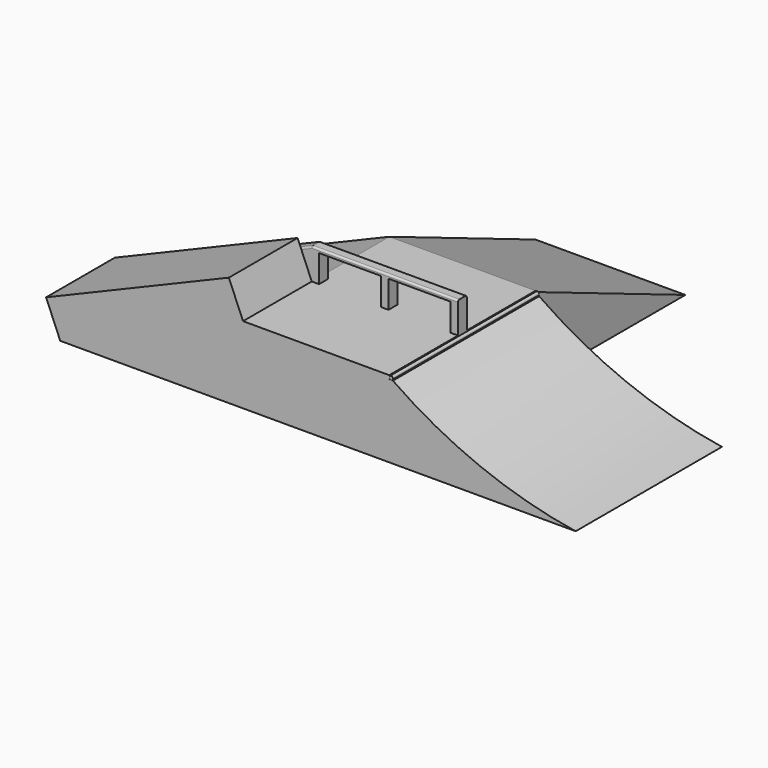
from build123d import *

# Parameters (mm, degrees)
F1_DEPTH     = 127
F2_W         = 5.08
F2_H         = 7.62
F3_DEPTH     = 19.05
F4_W         = 7.62
F4_H         = 2.54
F5_DEPTH     = 101.6
F6_T         = 5.08
F6_T3_DEPTH  = 17.78
F6_T5_DEPTH  = 15.24
F6_T7_DEPTH  = 15.24
F6_T9_DEPTH  = 15.24
F6_T11_DEPTH = 137.16
F8_DEPTH     = 7.62
F10_DEPTH    = 104.14
F11_R        = 1.27
F12_DEPTH    = 25.4


# Not quite as in the source:
# - a shell that OpenCascade refuses in one call is made with other operations: the cavity is built on its own and cut out
# - a feature names something its author has since deleted; it is built from what else it names


with BuildPart() as f1:
    # F0 (on Front) → F1 (new body)
    with BuildSketch(Plane.XZ):
        with BuildLine():
            Line((0, 50.8), (0, 0))
            Line((0, 0), (127, 0))
            ThreePointArc((127, 0), (60.6135499229, 18.1838748072), (0, 50.8))
        make_face()
        Polygon((-104.14, 0), (-2.54, 0), (-2.54, 50.8), (-2.54, 52.07), (-2.54, 53.34), (-104.14, 53.34), align=None)
        Polygon((-2.54, 0), (0, 0), (0, 50.8), (-1.27, 50.8), (-2.54, 50.8), align=None)
        Polygon((-231.14, 0), (-104.14, 0), (-104.14, 53.34), align=None)
    extrude(amount=F1_DEPTH)

    # F2 (on face) → F3 (join)
    with BuildSketch(Plane.XY.offset(53.34)):
        with Locations((-101.6, -63.5)):
            Rectangle(F2_W, F2_H)
        with Locations((-5.08, -63.5)):
            Rectangle(F2_W, F2_H)
        with Locations((-53.34, -63.5)):
            Rectangle(F2_W, F2_H)
    extrude(amount=F3_DEPTH)

    # F4 (on face) → F5 (join)
    with BuildSketch(Plane.YZ.offset(-2.54)):
        with Locations((-63.5, 73.66)):
            Rectangle(F4_W, F4_H)
    extrude(amount=-F5_DEPTH)

    # F6: shell of thickness 5.08, made by hand


with BuildPart() as f1b:
    # F0 (on Front) → F1, piece 2 (new body)
    with BuildSketch(Plane.XZ):
        with BuildLine():
            ThreePointArc((-2.54, 52.07), (-2.1680256121, 51.1719743879), (-1.27, 50.8))
            ThreePointArc((-1.27, 50.8), (-0.3719743879, 51.1719743879), (0, 52.07))
            ThreePointArc((0, 52.07), (-1.27, 53.34), (-2.54, 52.07))
        make_face()
    extrude(amount=F1_DEPTH)


with BuildPart() as f6_core1:
    # F6_t2: copy of F1
    add(f1.part)

    # the walls: a layer under each face that stays
    f6_faces = [f6_core1.faces().sort_by_distance(p)[0] for p in [
        (60.6135499229, -63.5, 18.1838748072),
        (-52.07, -127, 26.67),
        (-167.64, -63.5, 26.67),
        (-104.14, -63.5, 64.135),
        (-53.34, -67.31, 64.135),
        (-99.06, -63.5, 62.865),
        (-77.47, -63.5, 72.39),
        (-55.88, -63.5, 62.865),
        (-50.8, -63.5, 62.865),
        (-29.21, -63.5, 72.39),
        (-7.62, -63.5, 62.865),
        (-53.34, -63.5, 74.93),
        (-53.34, -59.69, 64.135),
        (-19.4733333333, -105.8333333333, 53.34),
        (-2.54, -63.5, 62.865),
        (-52.07, 0, 26.67),
        (-1.27, -63.5, 50.8),
    ]]
    thicken(f6_faces, amount=-F6_T, mode=Mode.SUBTRACT)

    # F6_s4 → F6_t3 (cut)
    with BuildSketch(Plane.XZ.offset(54.61)):
        Polygon((-104.2104714102, 53.386836691), (-102.1728589795, 48.6563309035), (-99.06, 49.9637316749), (-99.06, 53.34), align=None)
        Polygon((-99.0092, 53.3908), (-104.14, 53.34), (-104.14, 48.26), (-99.06, 48.26), align=None)
        Polygon((-99.0092, 72.3392), (-104.14, 72.39), (-104.14, 77.47), (-99.06, 77.47), align=None)
        Polygon((-55.9308, 72.3392), (-55.88, 77.47), (-50.8, 77.47), (-50.8, 72.39), align=None)
        Polygon((-55.9308, 53.3908), (-50.8, 53.34), (-50.8, 48.26), (-55.88, 48.26), align=None)
        Polygon((-50.7492, 53.3908), (-55.88, 53.34), (-55.88, 48.26), (-50.8, 48.26), align=None)
        Polygon((-50.7492, 72.3392), (-55.88, 72.39), (-55.88, 77.47), (-50.8, 77.47), align=None)
        Polygon((-7.6708, 72.3392), (-7.62, 77.47), (-2.54, 77.47), (-2.54, 72.39), align=None)
        Polygon((-7.6708, 53.3908), (-2.54, 53.34), (-2.54, 48.26), (-7.62, 48.26), align=None)
    extrude(amount=F6_T3_DEPTH, mode=Mode.SUBTRACT)

    # F6_s6 → F6_t5 (cut)
    with BuildSketch(Plane.YZ.offset(-60.96)):
        Polygon((-67.3608, 53.3908), (-62.23, 53.34), (-62.23, 48.26), (-67.31, 48.26), align=None)
        Polygon((-59.6392, 53.3908), (-64.77, 53.34), (-64.77, 48.26), (-59.69, 48.26), align=None)
    extrude(amount=F6_T5_DEPTH, mode=Mode.SUBTRACT)

    # F6_s8 → F6_t7 (cut)
    with BuildSketch(Plane.YZ.offset(-109.22)):
        Polygon((-67.3608, 53.3908), (-62.23, 53.34), (-62.23, 48.26), (-67.31, 48.26), align=None)
        Polygon((-59.6392, 53.3908), (-64.77, 53.34), (-64.77, 48.26), (-59.69, 48.26), align=None)
    extrude(amount=F6_T7_DEPTH, mode=Mode.SUBTRACT)

    # F6_s10 → F6_t9 (cut)
    with BuildSketch(Plane.YZ.offset(-12.7)):
        Polygon((-67.3608, 53.3908), (-62.23, 53.34), (-62.23, 48.26), (-67.31, 48.26), align=None)
        Polygon((-59.6392, 53.3908), (-64.77, 53.34), (-64.77, 48.26), (-59.69, 48.26), align=None)
    extrude(amount=F6_T9_DEPTH, mode=Mode.SUBTRACT)

    # F6_s12 → F6_t11 (cut)
    with BuildSketch(Plane.XZ.offset(-5.08)):
        Polygon((-2.4892, 50.8508), (-7.62, 50.8), (-7.62, 45.72), (-2.54, 45.72), align=None)
    extrude(amount=F6_T11_DEPTH, mode=Mode.SUBTRACT)


with BuildPart() as f1_1:
    add(f1.part)

    # what is left inside the walls is the cavity
    f6_cavity = [f6_core1.part.solids().sort_by_distance(p)[0] for p in [
        (-58.552758, -82.973333, 0.0508),
    ]]
    add(f6_cavity, mode=Mode.SUBTRACT)

    # F7 (on face) → F8 (join)
    with BuildSketch(Plane(origin=(0, -59.69, 0), x_dir=(-1, 0, 0), z_dir=(0, 1, 0))):
        Polygon((231.14, 21.59), (104.14, 74.93), (104.14, 53.34), (231.14, 0), align=None)
    extrude(amount=-F8_DEPTH)

    # F9 (on Right) → F10 (join)
    with BuildSketch(Plane.YZ):
        Polygon((127, 0), (0, 53.34), (0, 0), align=None)
    extrude(amount=-F10_DEPTH)

    # F11
    f11_edges = [f1_1.edges().sort_by_distance(p)[0] for p in [
        (-53.34, -67.31, 74.93),
        (-167.64, -67.31, 48.26),
        (-104.14, -63.5, 74.93),
        (-167.64, -59.69, 48.26),
        (-53.34, -59.69, 74.93),
    ]]
    fillet(f11_edges, radius=F11_R)

    # F12 (add): a face of the model
    f12_faces = [f1_1.faces().sort_by_distance(p)[0] for p in [
        (-167.64, -97.155, 26.67),
    ]]
    extrude(f12_faces, amount=F12_DEPTH)


solid = Compound([f1b.part, f1_1.part])
